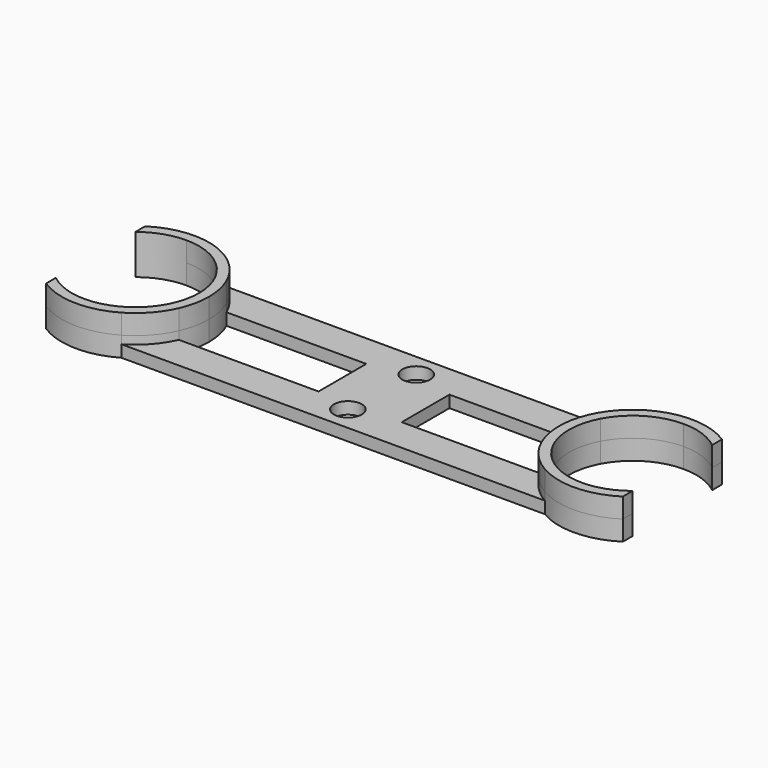
from build123d import *
from build123d import SkipClean  # not in build123d's __all__

# Parameters (mm, degrees)
F0_W     = 20.9095849469
F0_H     = 15
F1_DEPTH = 5
F2_DEPTH = 5
F3_R     = 3.5
F4_DEPTH = 2
F5_DEPTH = 5


# Not quite as in the source:
# - after a boolean that leaves OpenCascade's solid faulty, fix() repairs it


with BuildPart() as f1:
    # F0 (on Top) → F1 (new body)
    with BuildSketch(Plane.XY):
        with BuildLine():
            Line((-62.5, 16), (-53.2129121895, 16))
            ThreePointArc((-53.2129121895, 16), (-62.9177339073, 18.4952831388), (-72.5, 15.5643824163))
            Line((-72.5, 15.5643824163), (-72.5, 12.4899959968))
            ThreePointArc((-72.5, 12.4899959968), (-67.7990595416, 15.0970185128), (-62.5, 16))
        make_face()
        with BuildLine():
            ThreePointArc((-72.5, -15.5643824163), (-62.9177339073, -18.4952831388), (-53.2129121895, -16))
            Line((-53.2129121895, -16), (-62.5, -16))
            ThreePointArc((-62.5, -16), (-67.7990595416, -15.0970185128), (-72.5, -12.4899959968))
            Line((-72.5, -12.4899959968), (-72.5, -15.5643824163))
        make_face()
        with BuildLine():
            Line((-48.3667059749, 7.5), (-45.5884654747, 7.5))
            ThreePointArc((-45.5884654747, 7.5), (-48.7284912565, 12.3529570114), (-53.2129121895, 16))
            Line((-53.2129121895, 16), (-62.5, 16))
            ThreePointArc((-62.5, 16), (-54.2537887488, 13.7113092008), (-48.3667059749, 7.5))
        make_face()
        with BuildLine():
            ThreePointArc((-53.2129121895, -16), (-48.7284912565, -12.3529570114), (-45.5884654747, -7.5))
            Line((-45.5884654747, -7.5), (-48.3667059749, -7.5))
            ThreePointArc((-48.3667059749, -7.5), (-54.2537887488, -13.7113092008), (-62.5, -16))
            Line((-62.5, -16), (-53.2129121895, -16))
        make_face()
        with BuildLine():
            ThreePointArc((-44, 0), (-44.4014725914, 3.8331847909), (-45.5884654747, 7.5))
            Line((-45.5884654747, 7.5), (-48.3667059749, 7.5))
            ThreePointArc((-48.3667059749, 7.5), (-46.9736883903, 3.86440782), (-46.5, 0))
            ThreePointArc((-46.5, 0), (-46.9736883903, -3.86440782), (-48.3667059749, -7.5))
            Line((-48.3667059749, -7.5), (-45.5884654747, -7.5))
            ThreePointArc((-45.5884654747, -7.5), (-44.4014725914, -3.8331847909), (-44, 0))
        make_face()
        with BuildLine():
            ThreePointArc((-72.5, -15.5643824163), (-62.9177339073, -18.4952831388), (-53.2129121895, -16))
            Line((-53.2129121895, -16), (-62.5, -16))
            ThreePointArc((-62.5, -16), (-67.7990595416, -15.0970185128), (-72.5, -12.4899959968))
            Line((-72.5, -12.4899959968), (-72.5, -15.5643824163))
        make_face()
        with BuildLine():
            Line((-62.5, 16), (-53.2129121895, 16))
            ThreePointArc((-53.2129121895, 16), (-62.9177339073, 18.4952831388), (-72.5, 15.5643824163))
            Line((-72.5, 15.5643824163), (-72.5, 12.4899959968))
            ThreePointArc((-72.5, 12.4899959968), (-67.7990595416, 15.0970185128), (-62.5, 16))
        make_face()
        with BuildLine():
            ThreePointArc((72.5, 15.5643824163), (62.9177339073, 18.4952831388), (53.2129121895, 16))
            Line((53.2129121895, 16), (62.5, 16))
            ThreePointArc((62.5, 16), (67.7990595416, 15.0970185128), (72.5, 12.4899959968))
            Line((72.5, 12.4899959968), (72.5, 15.5643824163))
        make_face()
        with BuildLine():
            ThreePointArc((72.5, 15.5643824163), (62.9177339073, 18.4952831388), (53.2129121895, 16))
            Line((53.2129121895, 16), (62.5, 16))
            ThreePointArc((62.5, 16), (67.7990595416, 15.0970185128), (72.5, 12.4899959968))
            Line((72.5, 12.4899959968), (72.5, 15.5643824163))
        make_face()
        with BuildLine():
            Line((62.5, -16), (53.2129121895, -16))
            ThreePointArc((53.2129121895, -16), (62.9177339073, -18.4952831388), (72.5, -15.5643824163))
            Line((72.5, -15.5643824163), (72.5, -12.4899959968))
            ThreePointArc((72.5, -12.4899959968), (67.7990595416, -15.0970185128), (62.5, -16))
        make_face()
        with BuildLine():
            ThreePointArc((53.2129121895, 16), (48.7284912565, 12.3529570114), (45.5884654747, 7.5))
            Line((45.5884654747, 7.5), (48.3667059749, 7.5))
            ThreePointArc((48.3667059749, 7.5), (54.2537887488, 13.7113092008), (62.5, 16))
            Line((62.5, 16), (53.2129121895, 16))
        make_face()
        with BuildLine():
            Line((48.3667059749, 7.5), (45.5884654747, 7.5))
            ThreePointArc((45.5884654747, 7.5), (44, 0), (45.5884654747, -7.5))
            Line((45.5884654747, -7.5), (48.3667059749, -7.5))
            ThreePointArc((48.3667059749, -7.5), (46.5, 0), (48.3667059749, 7.5))
        make_face()
        with BuildLine():
            Line((48.3667059749, -7.5), (45.5884654747, -7.5))
            ThreePointArc((45.5884654747, -7.5), (48.7284912565, -12.3529570114), (53.2129121895, -16))
            Line((53.2129121895, -16), (62.5, -16))
            ThreePointArc((62.5, -16), (54.2537887488, -13.7113092008), (48.3667059749, -7.5))
        make_face()
        with BuildLine():
            Line((62.5, -16), (53.2129121895, -16))
            ThreePointArc((53.2129121895, -16), (62.9177339073, -18.4952831388), (72.5, -15.5643824163))
            Line((72.5, -15.5643824163), (72.5, -12.4899959968))
            ThreePointArc((72.5, -12.4899959968), (67.7990595416, -15.0970185128), (62.5, -16))
        make_face()
        with BuildLine():
            Line((10.4547924735, -7.5), (-10.4547924735, -7.5))
            Line((-10.4547924735, -7.5), (-45.5884654747, -7.5))
            ThreePointArc((-45.5884654747, -7.5), (-48.7284912565, -12.3529570114), (-53.2129121895, -16))
            Line((-53.2129121895, -16), (53.2129121895, -16))
            ThreePointArc((53.2129121895, -16), (48.7284912565, -12.3529570114), (45.5884654747, -7.5))
            Line((45.5884654747, -7.5), (10.4547924735, -7.5))
        make_face()
        with BuildLine():
            Line((-45.5884654747, 7.5), (-10.4547924735, 7.5))
            Line((-10.4547924735, 7.5), (10.4547924735, 7.5))
            Line((10.4547924735, 7.5), (45.5884654747, 7.5))
            ThreePointArc((45.5884654747, 7.5), (48.7284912565, 12.3529570114), (53.2129121895, 16))
            Line((53.2129121895, 16), (-53.2129121895, 16))
            ThreePointArc((-53.2129121895, 16), (-48.7284912565, 12.3529570114), (-45.5884654747, 7.5))
        make_face()
        Rectangle(F0_W, F0_H)
    extrude(amount=-F1_DEPTH)

    # F0 (on Top) → F2 (join)
    with BuildSketch(Plane.XY):
        with BuildLine():
            Line((-62.5, 16), (-53.2129121895, 16))
            ThreePointArc((-53.2129121895, 16), (-62.9177339073, 18.4952831388), (-72.5, 15.5643824163))
            Line((-72.5, 15.5643824163), (-72.5, 12.4899959968))
            ThreePointArc((-72.5, 12.4899959968), (-67.7990595416, 15.0970185128), (-62.5, 16))
        make_face()
        with BuildLine():
            ThreePointArc((-72.5, -15.5643824163), (-62.9177339073, -18.4952831388), (-53.2129121895, -16))
            Line((-53.2129121895, -16), (-62.5, -16))
            ThreePointArc((-62.5, -16), (-67.7990595416, -15.0970185128), (-72.5, -12.4899959968))
            Line((-72.5, -12.4899959968), (-72.5, -15.5643824163))
        make_face()
        with BuildLine():
            Line((-48.3667059749, 7.5), (-45.5884654747, 7.5))
            ThreePointArc((-45.5884654747, 7.5), (-48.7284912565, 12.3529570114), (-53.2129121895, 16))
            Line((-53.2129121895, 16), (-62.5, 16))
            ThreePointArc((-62.5, 16), (-54.2537887488, 13.7113092008), (-48.3667059749, 7.5))
        make_face()
        with BuildLine():
            ThreePointArc((-53.2129121895, -16), (-48.7284912565, -12.3529570114), (-45.5884654747, -7.5))
            Line((-45.5884654747, -7.5), (-48.3667059749, -7.5))
            ThreePointArc((-48.3667059749, -7.5), (-54.2537887488, -13.7113092008), (-62.5, -16))
            Line((-62.5, -16), (-53.2129121895, -16))
        make_face()
        with BuildLine():
            ThreePointArc((-44, 0), (-44.4014725914, 3.8331847909), (-45.5884654747, 7.5))
            Line((-45.5884654747, 7.5), (-48.3667059749, 7.5))
            ThreePointArc((-48.3667059749, 7.5), (-46.9736883903, 3.86440782), (-46.5, 0))
            ThreePointArc((-46.5, 0), (-46.9736883903, -3.86440782), (-48.3667059749, -7.5))
            Line((-48.3667059749, -7.5), (-45.5884654747, -7.5))
            ThreePointArc((-45.5884654747, -7.5), (-44.4014725914, -3.8331847909), (-44, 0))
        make_face()
        with BuildLine():
            Line((-62.5, 16), (-53.2129121895, 16))
            ThreePointArc((-53.2129121895, 16), (-62.9177339073, 18.4952831388), (-72.5, 15.5643824163))
            Line((-72.5, 15.5643824163), (-72.5, 12.4899959968))
            ThreePointArc((-72.5, 12.4899959968), (-67.7990595416, 15.0970185128), (-62.5, 16))
        make_face()
        with BuildLine():
            ThreePointArc((-72.5, -15.5643824163), (-62.9177339073, -18.4952831388), (-53.2129121895, -16))
            Line((-53.2129121895, -16), (-62.5, -16))
            ThreePointArc((-62.5, -16), (-67.7990595416, -15.0970185128), (-72.5, -12.4899959968))
            Line((-72.5, -12.4899959968), (-72.5, -15.5643824163))
        make_face()
        with BuildLine():
            Line((62.5, -16), (53.2129121895, -16))
            ThreePointArc((53.2129121895, -16), (62.9177339073, -18.4952831388), (72.5, -15.5643824163))
            Line((72.5, -15.5643824163), (72.5, -12.4899959968))
            ThreePointArc((72.5, -12.4899959968), (67.7990595416, -15.0970185128), (62.5, -16))
        make_face()
        with BuildLine():
            ThreePointArc((72.5, 15.5643824163), (62.9177339073, 18.4952831388), (53.2129121895, 16))
            Line((53.2129121895, 16), (62.5, 16))
            ThreePointArc((62.5, 16), (67.7990595416, 15.0970185128), (72.5, 12.4899959968))
            Line((72.5, 12.4899959968), (72.5, 15.5643824163))
        make_face()
        with BuildLine():
            Line((62.5, -16), (53.2129121895, -16))
            ThreePointArc((53.2129121895, -16), (62.9177339073, -18.4952831388), (72.5, -15.5643824163))
            Line((72.5, -15.5643824163), (72.5, -12.4899959968))
            ThreePointArc((72.5, -12.4899959968), (67.7990595416, -15.0970185128), (62.5, -16))
        make_face()
        with BuildLine():
            ThreePointArc((53.2129121895, 16), (48.7284912565, 12.3529570114), (45.5884654747, 7.5))
            Line((45.5884654747, 7.5), (48.3667059749, 7.5))
            ThreePointArc((48.3667059749, 7.5), (54.2537887488, 13.7113092008), (62.5, 16))
            Line((62.5, 16), (53.2129121895, 16))
        make_face()
        with BuildLine():
            Line((48.3667059749, 7.5), (45.5884654747, 7.5))
            ThreePointArc((45.5884654747, 7.5), (44, 0), (45.5884654747, -7.5))
            Line((45.5884654747, -7.5), (48.3667059749, -7.5))
            ThreePointArc((48.3667059749, -7.5), (46.5, 0), (48.3667059749, 7.5))
        make_face()
        with BuildLine():
            Line((48.3667059749, -7.5), (45.5884654747, -7.5))
            ThreePointArc((45.5884654747, -7.5), (48.7284912565, -12.3529570114), (53.2129121895, -16))
            Line((53.2129121895, -16), (62.5, -16))
            ThreePointArc((62.5, -16), (54.2537887488, -13.7113092008), (48.3667059749, -7.5))
        make_face()
        with BuildLine():
            ThreePointArc((72.5, 15.5643824163), (62.9177339073, 18.4952831388), (53.2129121895, 16))
            Line((53.2129121895, 16), (62.5, 16))
            ThreePointArc((62.5, 16), (67.7990595416, 15.0970185128), (72.5, 12.4899959968))
            Line((72.5, 12.4899959968), (72.5, 15.5643824163))
        make_face()
    extrude(amount=F2_DEPTH)

    # F3 (on face) → F4 (cut)
    with BuildSketch(Plane.XY):
        with BuildLine():
            ThreePointArc((45.5884654747, 7.5), (48.7284912565, 12.3529570114), (53.2129121895, 16))
            Line((53.2129121895, 16), (-53.2129121895, 16))
            ThreePointArc((-53.2129121895, 16), (-48.7284912565, 12.3529570114), (-45.5884654747, 7.5))
            Line((-45.5884654747, 7.5), (-10.4547924735, 7.5))
            Line((-10.4547924735, 7.5), (-10.4547924735, -7.5))
            Line((-10.4547924735, -7.5), (-45.5884654747, -7.5))
            ThreePointArc((-45.5884654747, -7.5), (-48.7284912565, -12.3529570114), (-53.2129121895, -16))
            Line((-53.2129121895, -16), (53.2129121895, -16))
            ThreePointArc((53.2129121895, -16), (48.7284912565, -12.3529570114), (45.5884654747, -7.5))
            Line((45.5884654747, -7.5), (10.4547924735, -7.5))
            Line((10.4547924735, -7.5), (10.4547924735, 7.5))
            Line((10.4547924735, 7.5), (45.5884654747, 7.5))
        make_face()
        with Locations((-1.2, -9.8506268114)):
            Circle(F3_R, mode=Mode.SUBTRACT)
        with Locations((0, 10.1133407302)):
            Circle(F3_R, mode=Mode.SUBTRACT)
        with BuildLine():
            ThreePointArc((45.5884654747, 7.5), (48.7284912565, 12.3529570114), (53.2129121895, 16))
            Line((53.2129121895, 16), (-53.2129121895, 16))
            ThreePointArc((-53.2129121895, 16), (-48.7284912565, 12.3529570114), (-45.5884654747, 7.5))
            Line((-45.5884654747, 7.5), (-10.4547924735, 7.5))
            Line((-10.4547924735, 7.5), (-10.4547924735, -7.5))
            Line((-10.4547924735, -7.5), (-45.5884654747, -7.5))
            ThreePointArc((-45.5884654747, -7.5), (-48.7284912565, -12.3529570114), (-53.2129121895, -16))
            Line((-53.2129121895, -16), (53.2129121895, -16))
            ThreePointArc((53.2129121895, -16), (48.7284912565, -12.3529570114), (45.5884654747, -7.5))
            Line((45.5884654747, -7.5), (10.4547924735, -7.5))
            Line((10.4547924735, -7.5), (10.4547924735, 7.5))
            Line((10.4547924735, 7.5), (45.5884654747, 7.5))
        make_face()
        with Locations((-1.2, -9.8506268114)):
            Circle(F3_R, mode=Mode.SUBTRACT)
        with Locations((0, 10.1133407302)):
            Circle(F3_R, mode=Mode.SUBTRACT)
    with SkipClean():  # cleaning this boolean's faces spoils the solid; the shape is the same uncleaned
        extrude(amount=-F4_DEPTH, mode=Mode.SUBTRACT)

    # F5 (cut, through all): faces of the model
    f5_faces = [f1.faces().sort_by_distance(p)[0] for p in [
        (0, 10.1133407302, 0),
        (-1.2, -9.8506268114, 0),
    ]]
    extrude(f5_faces, amount=-F5_DEPTH, mode=Mode.SUBTRACT)

    add(f1.part.fix(), mode=Mode.REPLACE)


solid = f1.part
